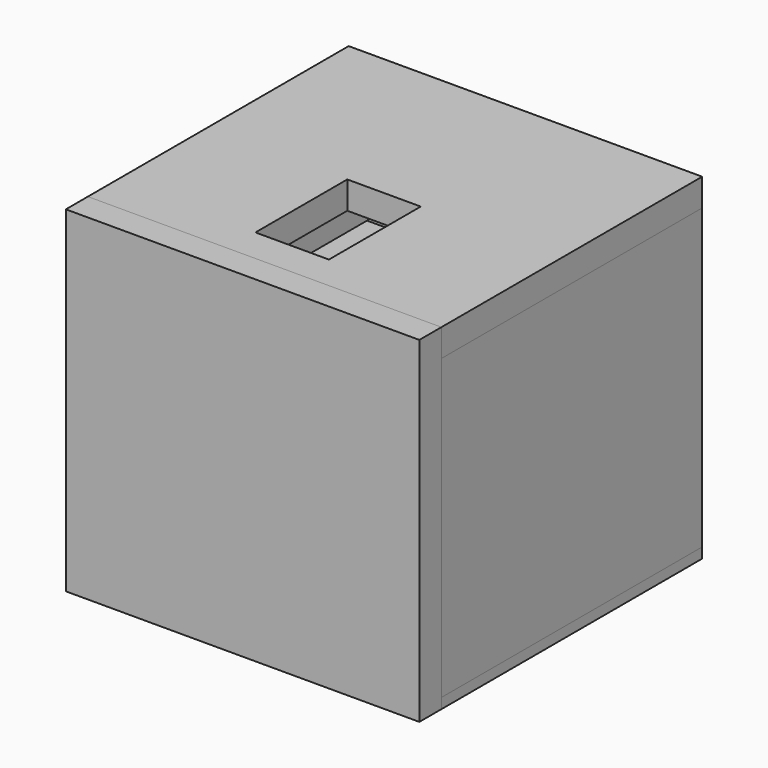
from build123d import *

# Parameters (mm, degrees)
F0_W      = 154
F0_H      = 146.5
F1_DEPTH  = 12
F2_W      = 142
F2_H      = 130
F3_DEPTH  = 12
F5_W      = 154
F5_H      = 142
F5_W_2    = 32
F5_H_2    = 50
F6_DEPTH  = 12
F7_W      = 154
F7_H      = 142
F8_DEPTH  = 4.5
F10_W     = 130
F10_H     = 130
F11_DEPTH = 4.5
F12_W     = 3
F12_H     = 3
F13_DEPTH = 142
F15_W     = 136
F15_H     = 137
F16_DEPTH = 3


# Not quite as in the source:
# - a feature names something its author has since deleted; it is built from what else it names


with BuildPart() as f1:
    # F0 (on Front) → F1 (new body)
    with BuildSketch(Plane.XZ):
        with Locations((0, 3.75)):
            Rectangle(F0_W, F0_H)
    extrude(amount=F1_DEPTH)


with BuildPart() as f3:
    # F2 (on face) → F3 (new body)
    with BuildSketch(Plane.YZ.offset(77)):
        with Locations((71, 0)):
            Rectangle(F2_W, F2_H)
    extrude(amount=-F3_DEPTH)

    # F12 (on face) → F13 (cut)
    with BuildSketch(Plane(origin=(0, 142, 0), x_dir=(-1, 0, 0), z_dir=(0, 1, 0))):
        with Locations((-66.5, 14.5)):
            Rectangle(F12_W, F12_H)
        with Locations((-66.5, -28.5)):
            Rectangle(F12_W, F12_H)
    extrude(amount=-F13_DEPTH, mode=Mode.SUBTRACT)


with BuildPart() as f4_1:
    # F4: instance of F1
    add(f1.part.mirror(Plane.YZ))


with BuildPart() as f6:
    # F5 (on face) → F6 (new body)
    with BuildSketch(Plane.XY.offset(77)):
        with Locations((0, 71)):
            Rectangle(F5_W, F5_H)
        with Locations((0, 40)):
            Rectangle(F5_W_2, F5_H_2, mode=Mode.SUBTRACT)
    extrude(amount=-F6_DEPTH)


with BuildPart() as f8:
    # F7 (on face) → F8 (new body)
    with BuildSketch(Plane(origin=(0, 0, -69.5), x_dir=(1, 0, 0), z_dir=(0, 0, -1))):
        with Locations((0, -71)):
            Rectangle(F7_W, F7_H)
    extrude(amount=-F8_DEPTH)


with BuildPart() as f11:
    # F10 (on face) → F11 (new body)
    with BuildSketch(Plane(origin=(0, 142, 0), x_dir=(-1, 0, 0), z_dir=(0, 1, 0))):
        Rectangle(F10_W, F10_H)
    extrude(amount=-F11_DEPTH)


with BuildPart() as f14_1:
    # F14: instance of F3
    add(f3.part.mirror(Plane.YZ))


with BuildPart() as f16:
    # F15 (on face) → F16 (new body)
    with BuildSketch(Plane.XY.offset(13)):
        with Locations((0, 68.5)):
            Rectangle(F15_W, F15_H)
    extrude(amount=F16_DEPTH)


with BuildPart() as f17_1:
    # F17: copy of F16
    add(f16.part.moved(Location((0, 0, -43))))


solid = Compound([f1.part, f3.part, f6.part, f8.part, f11.part, f14_1.part, f16.part, f17_1.part])
